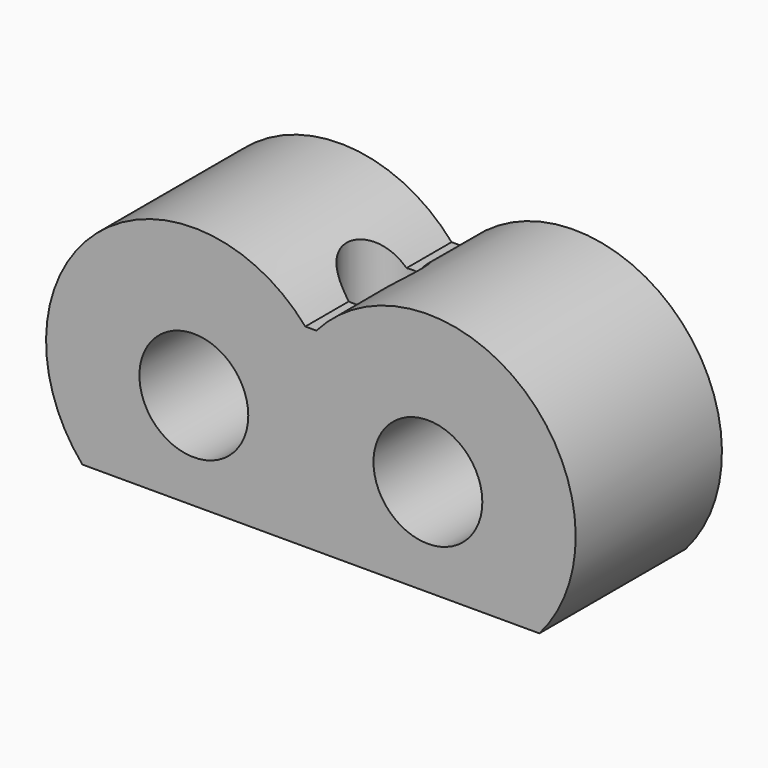
from build123d import *

# Parameters (mm, degrees)
F0_R           = 1.488728542
F1_DEPTH       = 5
F5_D           = 2
F5_CSINK_D     = 2.5
F5_CSINK_ANGLE = 90


# Not quite as in the source:
# - a feature of the source that left no trace in its solid (it failed there, or was rolled back) is left out


with BuildPart() as f1:
    # F0 (on Front) → F1 (new body)
    with BuildSketch(Plane.XZ):
        with BuildLine():
            Line((-6.25, -2.6532969418), (6.25, -2.6532969418))
            ThreePointArc((6.25, -2.6532969418), (5.854172537, 3.0491244048), (0.1517511904, 2.6532969418))
            Line((0.1517511904, 2.6532969418), (-0.1517511904, 2.6532969418))
            ThreePointArc((-0.1517511904, 2.6532969418), (-5.854172537, 3.0491244048), (-6.25, -2.6532969418))
        make_face()
        with Locations((-3.2008755952, 0)):
            Circle(F0_R, mode=Mode.SUBTRACT)
        with Locations((3.2008755952, 0)):
            Circle(F0_R, mode=Mode.SUBTRACT)
    extrude(amount=F1_DEPTH)

    # F5 (through all)
    with Locations(Plane(origin=(0, 0, -2.6532969418), x_dir=(1, 0, 0), z_dir=(0, 0, -1))):
        with Locations((0, 2.525947988)):
            CounterSinkHole(F5_D / 2, F5_CSINK_D / 2, counter_sink_angle=F5_CSINK_ANGLE)


solid = f1.part
